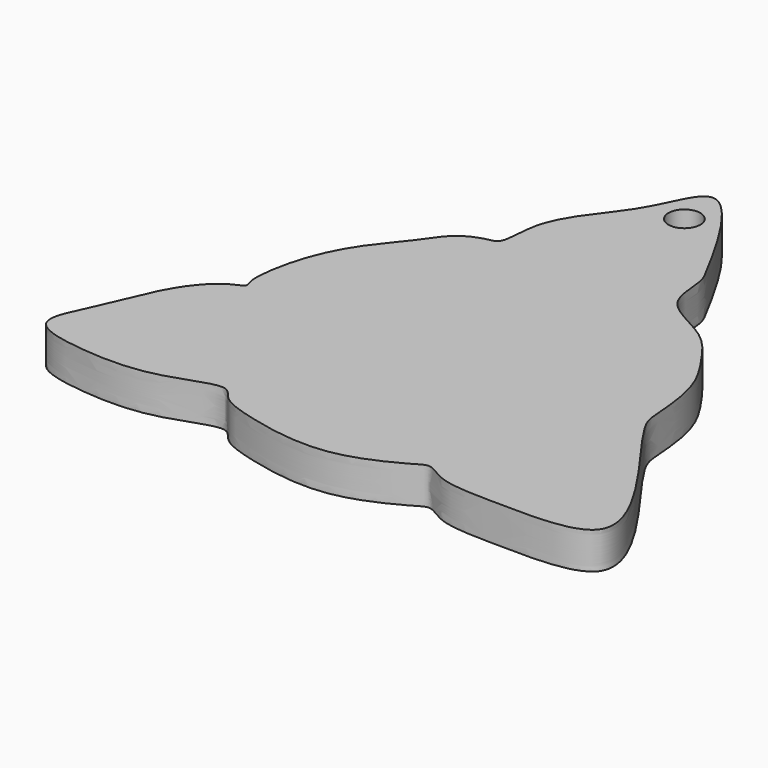
from build123d import *

# Parameters (mm, degrees)
F0_R      = 2.1677075124
F1_DEPTH  = 5
F22_DEPTH = 1


# Not quite as in the source:
# - the program builds the solid bodies; features that only make, move or delete a surface that nothing else refers to are left out


with BuildPart() as f1:
    # F0 (on Top) → F1 (new body)
    with BuildSketch(Plane.XY):
        with BuildLine():
            add(Edge.make_bspline(
                [(40.1755683124, 73.3752697706), (38.7738536908, 73.6329763294), (37.0397231233, 69.8078414808), (35.296300795, 66.4160600882), (33.0165298684, 63.3818863105), (28.5281579812, 57.54996442), (29.2080482989, 51.1260150857), (26.8750986244, 51.0479956768), (23.5913091085, 49.6059134152), (21.4609417314, 45.9744364473), (17.3522987297, 41.4461778552), (14.1947755243, 35.027557672), (13.1743465653, 28.0102457802), (14.2235529323, 26.5834728824), (11.96115391, 25.9660934767), (9.0178297831, 23.0585124898), (6.7531303526, 18.9063559913), (4.4176713861, 12.7402725008), (0.7019220994, 5.9245631673), (9.5555563077, 4.1114505526), (18.9399035673, 3.9355471624), (26.9834982739, 8.0214044539), (28.3615750008, 4.8528221744), (33.3823107874, 3.1442572994), (44.3591772545, 0.8802375496), (53.1308781915, 5.5731632508), (55.0919888579, 6.8870737383), (57.9471626601, 4.3480542693), (65.8747745815, 4.3041671001), (82.4806196859, 3.9811379019), (74.1793070499, 18.4737516588), (66.5429336412, 27.9091143572), (66.3137165708, 30.9533987516), (65.7485539565, 38.3704674859), (62.22374839, 43.571772342), (58.6910569926, 48.60994325), (50.948707278, 51.249168376), (51.2501021264, 57.4639921826), (49.554362213, 60.4654785603), (42.7794043821, 72.8965520468), (40.1755683124, 73.3752697706)],
                knots=[0, 0, 0, 0, 0.0230439272, 0.0453558062, 0.0664571143, 0.0963302943, 0.1219279647, 0.1359671901, 0.1560941129, 0.178390919, 0.2052153731, 0.2354584948, 0.2639004598, 0.275388064, 0.2898329647, 0.312069089, 0.3359058806, 0.3649949879, 0.3913929581, 0.419725118, 0.4553509393, 0.485521153, 0.5021076814, 0.526424317, 0.5635424468, 0.5972920276, 0.612162225, 0.6307961322, 0.6630510879, 0.7010873964, 0.7392599123, 0.7780867485, 0.7966686803, 0.8256207675, 0.8532656635, 0.8803382417, 0.9099311428, 0.9340949437, 0.9571934202, 1, 1, 1, 1], degree=3))
        make_face()
        with Locations((40.5923016369, 67.7139237523)):
            Circle(F0_R, mode=Mode.SUBTRACT)
    extrude(amount=F1_DEPTH)

    # F0 (on Top) → F22 (join)
    with BuildSketch(Plane.XY):
        with BuildLine():
            add(Edge.make_bspline(
                [(40.1755683124, 73.3752697706), (38.7738536908, 73.6329763294), (37.0397231233, 69.8078414808), (35.296300795, 66.4160600882), (33.0165298684, 63.3818863105), (28.5281579812, 57.54996442), (29.2080482989, 51.1260150857), (26.8750986244, 51.0479956768), (23.5913091085, 49.6059134152), (21.4609417314, 45.9744364473), (17.3522987297, 41.4461778552), (14.1947755243, 35.027557672), (13.1743465653, 28.0102457802), (14.2235529323, 26.5834728824), (11.96115391, 25.9660934767), (9.0178297831, 23.0585124898), (6.7531303526, 18.9063559913), (4.4176713861, 12.7402725008), (0.7019220994, 5.9245631673), (9.5555563077, 4.1114505526), (18.9399035673, 3.9355471624), (26.9834982739, 8.0214044539), (28.3615750008, 4.8528221744), (33.3823107874, 3.1442572994), (44.3591772545, 0.8802375496), (53.1308781915, 5.5731632508), (55.0919888579, 6.8870737383), (57.9471626601, 4.3480542693), (65.8747745815, 4.3041671001), (82.4806196859, 3.9811379019), (74.1793070499, 18.4737516588), (66.5429336412, 27.9091143572), (66.3137165708, 30.9533987516), (65.7485539565, 38.3704674859), (62.22374839, 43.571772342), (58.6910569926, 48.60994325), (50.948707278, 51.249168376), (51.2501021264, 57.4639921826), (49.554362213, 60.4654785603), (42.7794043821, 72.8965520468), (40.1755683124, 73.3752697706)],
                knots=[0, 0, 0, 0, 0.0230439272, 0.0453558062, 0.0664571143, 0.0963302943, 0.1219279647, 0.1359671901, 0.1560941129, 0.178390919, 0.2052153731, 0.2354584948, 0.2639004598, 0.275388064, 0.2898329647, 0.312069089, 0.3359058806, 0.3649949879, 0.3913929581, 0.419725118, 0.4553509393, 0.485521153, 0.5021076814, 0.526424317, 0.5635424468, 0.5972920276, 0.612162225, 0.6307961322, 0.6630510879, 0.7010873964, 0.7392599123, 0.7780867485, 0.7966686803, 0.8256207675, 0.8532656635, 0.8803382417, 0.9099311428, 0.9340949437, 0.9571934202, 1, 1, 1, 1], degree=3))
        make_face()
        with Locations((40.5923016369, 67.7139237523)):
            Circle(F0_R, mode=Mode.SUBTRACT)
    extrude(amount=F22_DEPTH)


solid = f1.part
